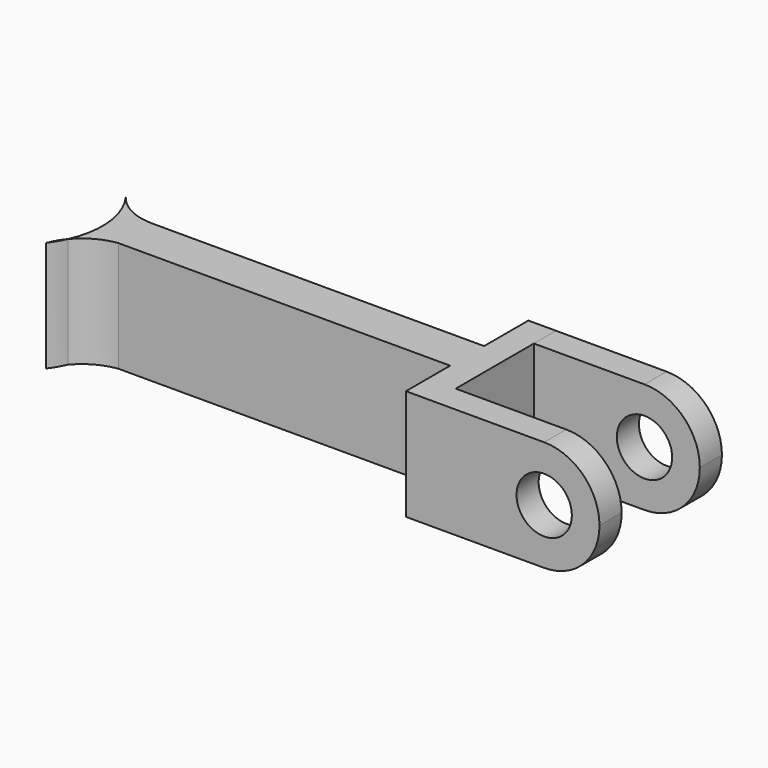
from build123d import *
from build123d import SkipClean  # not in build123d's __all__

# Parameters (mm, degrees)
F1_DEPTH = 2
F3_DEPTH = 0.5
F5_DEPTH = 0.5
F6_R     = 0.5
F7_DEPTH = 25


# Not quite as in the source:
# - a pattern or mirror of a feature is missing from the dataset's text; its kind, count and spacing are read off the source's solid


with BuildPart() as f1:
    # F0 (on Top) → F1 (new body)
    with BuildSketch(Plane.XY):
        with BuildLine():
            ThreePointArc((2.399318749, 16.9524586827), (2.4914108716, 17.0905545243), (2.5676812283, 17.23797994))
            ThreePointArc((2.5676812283, 17.23797994), (2.4715876211, 17.1022436421), (2.399318749, 16.9524586827))
        make_face()
    extrude(amount=F1_DEPTH)


with BuildPart() as f1b:
    # F0 (on Top) → F1, piece 2 (new body)
    with BuildSketch(Plane.XY):
        with BuildLine():
            ThreePointArc((3.199318749, 18.3524586827), (2.7521051535, 18.4580314917), (2.399318749, 18.7524586827))
            ThreePointArc((2.399318749, 18.7524586827), (2.6901349421, 18.0181906296), (2.5676812283, 17.23797994))
            ThreePointArc((2.5676812283, 17.23797994), (2.8511129134, 17.4705505548), (3.199318749, 17.5853342952))
            Line((3.199318749, 17.5853342952), (9.199318749, 17.5853342952))
            Line((9.199318749, 17.5853342952), (9.199318749, 16.5853342952))
            Line((9.199318749, 16.5853342952), (11.699318749, 16.5853342952))
            Line((11.699318749, 16.5853342952), (11.699318749, 17.0853342952))
            Line((11.699318749, 17.0853342952), (9.699318749, 17.0853342952))
            Line((9.699318749, 17.0853342952), (9.699318749, 18.8524586827))
            Line((9.699318749, 18.8524586827), (11.699318749, 18.8524586827))
            Line((11.699318749, 18.8524586827), (11.699318749, 19.3524586827))
            Line((11.699318749, 19.3524586827), (9.199318749, 19.3524586827))
            Line((9.199318749, 19.3524586827), (9.199318749, 18.3524586827))
            Line((9.199318749, 18.3524586827), (3.199318749, 18.3524586827))
        make_face()
    extrude(amount=F1_DEPTH)

    # F2 (on face) → F3 (join)
    with BuildSketch(Plane.XZ.offset(-16.5853342952)):
        with BuildLine():
            ThreePointArc((11.699318749, 0), (12.4064255302, 0.2928932188), (12.699318749, 1))
            ThreePointArc((12.699318749, 1), (12.4064255302, 1.7071067812), (11.699318749, 2))
            Line((11.699318749, 2), (11.699318749, 0))
        make_face()
        with BuildLine():
            Line((11.699318749, 0), (11.699318749, 2))
            ThreePointArc((11.699318749, 2), (10.699318749, 1), (11.699318749, 0))
        make_face()
        with BuildLine():
            ThreePointArc((11.699318749, 0), (10.699318749, 1), (11.699318749, 2))
            Line((11.699318749, 2), (9.699318749, 2))
            Line((9.699318749, 2), (9.699318749, 0))
            Line((9.699318749, 0), (11.699318749, 0))
        make_face()
    f3 = extrude(amount=-F3_DEPTH)

    # F3_copies: F3 across plane
    with SkipClean():  # cleaning this boolean's faces spoils the solid; the shape is the same uncleaned
        add(f3.mirror(Plane.ZX.offset(17.968896)), clean=False)

    # F4 (on face) → F5 (join)
    with BuildSketch(Plane.XZ.offset(-18.8524586827)):
        with BuildLine():
            Line((11.699318749, 0), (11.699318749, 2))
            ThreePointArc((11.699318749, 2), (10.699318749, 1), (11.699318749, 0))
        make_face()
    with SkipClean():  # cleaning this boolean's faces spoils the solid; the shape is the same uncleaned
        extrude(amount=-F5_DEPTH)

    # F6 (on face) → F7 (cut)
    with BuildSketch(Plane.XZ.offset(-16.5853342952)):
        with Locations((11.699318749, 1)):
            Circle(F6_R)
    with SkipClean():  # cleaning this boolean's faces spoils the solid; the shape is the same uncleaned
        extrude(amount=-F7_DEPTH, mode=Mode.SUBTRACT)


solid = Compound([f1.part, f1b.part])
